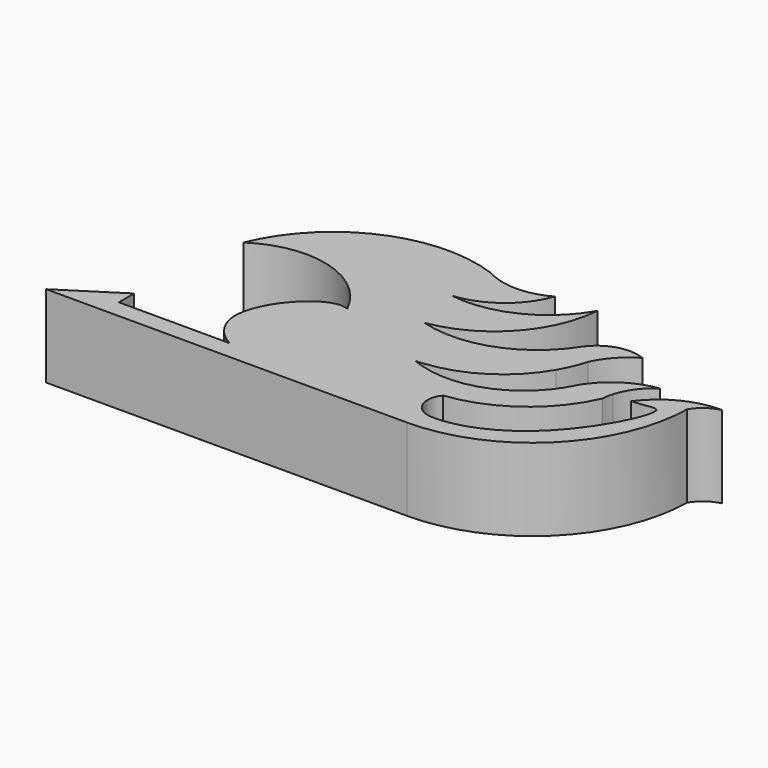
from build123d import *

# Parameters (mm, degrees)
F1_DEPTH = 25.4


with BuildPart() as f1:
    # F0 (on Top) → F1 (new body)
    with BuildSketch(Plane.XY):
        with BuildLine():
            add(Edge.make_bspline(
                [(-26.2610681984, -10.8273644), (-22.3250154222, -12.9399033802), (-6.7541943176, -14.1664240285), (-7.861061568, 17.5830890308), (-15.3270475566, 20.9516510367)],
                knots=[0.4911658302, 0.4911658302, 0.4911658302, 0.4911658302, 0.6402639099, 1, 1, 1, 1], degree=3))
            add(Edge.make_bspline(
                [(-15.3270475566, 20.9516510367), (-22.3564971203, 24.123253121), (-41.1418845104, 4.1977350509), (-30.2859655215, -8.6671412095), (-26.2610681984, -10.8273644)],
                knots=[0, 0, 0, 0, 0.3387023101, 0.4911658302, 0.4911658302, 0.4911658302, 0.4911658302], degree=3))
        make_face()
        with BuildLine():
            add(Edge.make_bspline(
                [(35.5182294418, -10.447258051), (31.9129186826, -10.220612291), (23.1955555043, -7.2820451281), (18.0529932429, 2.8715139484), (17.1729191086, 8.9899072036)],
                knots=[0.4660645619, 0.4660645619, 0.4660645619, 0.4660645619, 0.5346510085, 0.6442786993, 0.6442786993, 0.6442786993, 0.6442786993], degree=3))
            ThreePointArc((35.5182294418, -10.447258051), (30.0729748302, -6.5945561838), (31.0759395361, 0))
            ThreePointArc((31.0759395361, 0), (49.5151308357, 7.2590451113), (62.0112679899, 22.6390343159))
            ThreePointArc((62.0112679899, 22.6390343159), (62.2358256831, 24.395139963), (62.6415775007, 26.1184213282))
            add(Edge.make_bspline(
                [(54.4754700357, 26.7574300255), (57.3752815642, 26.5086516013), (60.1433747449, 26.2647226636), (62.6415775007, 26.1184213282)],
                knots=[0.9219128776, 0.9219128776, 0.9219128776, 0.9219128776, 0.9641346796, 0.9641346796, 0.9641346796, 0.9641346796], degree=3))
            ThreePointArc((54.4754700357, 26.7574300255), (53.7133787969, 25.7031684966), (53.0118979514, 24.6076434851))
            ThreePointArc((53.0118979514, 24.6076434851), (38.016967787, 10.0876095615), (17.1729191086, 8.9899072036))
        make_face()
        with BuildLine():
            ThreePointArc((-56.50515552, 32.3630547615), (-33.3182753375, 36.0316218628), (-15.3270475566, 20.9516510367))
            add(Edge.make_bspline(
                [(-26.2610681984, -10.8273644), (-22.3250154222, -12.9399033802), (-6.7541943176, -14.1664240285), (-7.861061568, 17.5830890308), (-15.3270475566, 20.9516510367)],
                knots=[0.4911658302, 0.4911658302, 0.4911658302, 0.4911658302, 0.6402639099, 1, 1, 1, 1], degree=3))
            Line((-26.2610681984, -10.8273644), (-60.464620338, -10.8273644))
            Line((-60.464620338, -10.8273644), (-60.464620338, -4.9215289764))
            Line((-60.464620338, -4.9215289764), (-78.4632340074, -16.4519678801))
            Line((-78.4632340074, -16.4519678801), (-14.9052012712, -16.4519678801))
            Line((-14.9052012712, -16.4519678801), (33.0445505679, -16.4519678801))
            ThreePointArc((33.0445505679, -16.4519678801), (67.0192612888, -2.5629170358), (81.5344079335, 31.1490573918))
            ThreePointArc((81.5344079335, 31.1490573918), (84.4106855525, 34.3353672495), (88.3062928915, 36.1380837858))
            ThreePointArc((88.3062928915, 36.1380837858), (77.0854781582, 33.5158631028), (68.3389529586, 26.0137952864))
            add(Edge.make_bspline(
                [(68.3389529586, 26.0137952864), (73.13500471, 26.2276507448), (80.3696253608, 30.0761350301), (65.6763095341, -1.3650666606), (43.6762193769, -10.9601053344), (35.5182294418, -10.447258051)],
                knots=[0, 0, 0, 0, 0.1043811632, 0.3108691907, 0.4660645619, 0.4660645619, 0.4660645619, 0.4660645619], degree=3))
            add(Edge.make_bspline(
                [(35.5182294418, -10.447258051), (31.9129186826, -10.220612291), (23.1955555043, -7.2820451281), (18.0529932429, 2.8715139484), (17.1729191086, 8.9899072036)],
                knots=[0.4660645619, 0.4660645619, 0.4660645619, 0.4660645619, 0.5346510085, 0.6442786993, 0.6442786993, 0.6442786993, 0.6442786993], degree=3))
            ThreePointArc((17.1729191086, 8.9899072036), (15.8161613784, 9.4543765839), (14.4833568484, 9.9836736917))
            ThreePointArc((14.4833568484, 9.9836736917), (15.7599932562, 10.0425488454), (17.0336540583, 10.1476914274))
            add(Edge.make_bspline(
                [(17.0336540583, 10.1476914274), (16.5524367293, 15.1345962527), (19.2361600934, 26.9166935874), (34.5605586177, 27.9160004318), (43.9602541666, 27.5027224979)],
                knots=[0.6512070875, 0.6512070875, 0.6512070875, 0.6512070875, 0.7409649976, 0.872432959, 0.872432959, 0.872432959, 0.872432959], degree=3))
            ThreePointArc((43.9602541666, 27.5027224979), (45.9259805238, 31.4321090753), (47.3872944713, 35.5756245553))
            ThreePointArc((47.3872944713, 35.5756245553), (51.1063153143, 41.2109006624), (56.3866607845, 45.4186797142))
            ThreePointArc((56.3866607845, 45.4186797142), (48.2264153253, 45.809802792), (41.481461376, 41.2002280354))
            ThreePointArc((41.481461376, 41.2002280354), (25.0576689955, 27.6740129875), (3.7966074888, 26.8574878573))
            ThreePointArc((3.7966074888, 26.8574878573), (23.5274065425, 37.3289516325), (32.4820913374, 57.7928125858))
            ThreePointArc((32.4820913374, 57.7928125858), (18.6619239349, 44.9253049217), (0, 42.0439206064))
            ThreePointArc((0, 42.0439206064), (12.1179065959, 46.7589869992), (19.8267325759, 57.2303533554))
            ThreePointArc((19.8267325759, 57.2303533554), (9.9133662879, 54.6642939776), (0, 57.2303533554))
            ThreePointArc((0, 57.2303533554), (-33.2620682112, 56.1796066262), (-56.50515552, 32.3630547615))
        make_face()
        with BuildLine():
            ThreePointArc((17.0336540583, 10.1476914274), (32.5838091219, 15.5874190212), (43.9602541666, 27.5027224979))
            add(Edge.make_bspline(
                [(17.0336540583, 10.1476914274), (16.5524367293, 15.1345962527), (19.2361600934, 26.9166935874), (34.5605586177, 27.9160004318), (43.9602541666, 27.5027224979)],
                knots=[0.6512070875, 0.6512070875, 0.6512070875, 0.6512070875, 0.7409649976, 0.872432959, 0.872432959, 0.872432959, 0.872432959], degree=3))
        make_face()
        with BuildLine():
            add(Edge.make_bspline(
                [(54.4754700357, 26.7574300255), (57.3752815642, 26.5086516013), (60.1433747449, 26.2647226636), (62.6415775007, 26.1184213282)],
                knots=[0.9219128776, 0.9219128776, 0.9219128776, 0.9219128776, 0.9641346796, 0.9641346796, 0.9641346796, 0.9641346796], degree=3))
            ThreePointArc((62.6415775007, 26.1184213282), (65.2892454144, 31.4686261622), (69.6213813016, 35.5756245553))
            ThreePointArc((69.6213813016, 35.5756245553), (61.1788209316, 32.6601387253), (54.4754700357, 26.7574300255))
        make_face()
    extrude(amount=F1_DEPTH)


solid = f1.part
